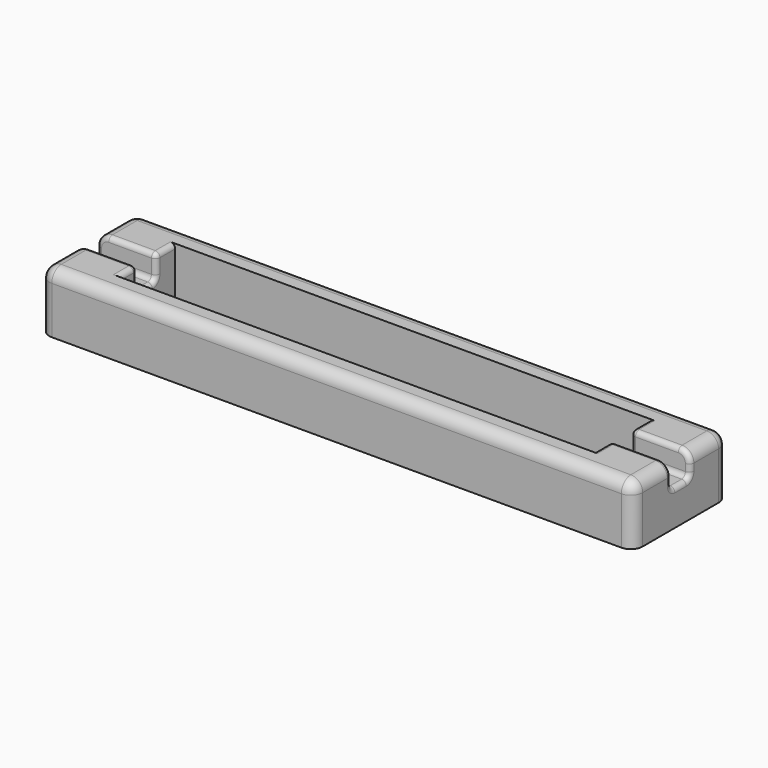
from build123d import *

# Parameters (mm, degrees)
F0_W         = 25
F0_H         = 5
F1_DEPTH     = 2.5
F2_W         = 20
F2_H         = 3
F3_DEPTH     = 2
F4_W         = 2.5
F4_H         = 1
F5_DEPTH     = 1
F6_F1_R      = 0.2
F6_F2_R      = 0.2
F7_T1_DEPTH  = 24
F7_T3_DEPTH  = 1.5
F7_T5_DEPTH  = 3.25
F7_T7_DEPTH  = 1.5
F7_T10_ANGLE = 90
F7_T12_ANGLE = 90
F7_T14_ANGLE = 90
F7_T16_ANGLE = 90
F7_S19_W     = 0.5
F7_S19_H     = 0.5
F7_T20_DEPTH = 0.5
F7_S25_W     = 0.5
F7_S25_H     = 0.5
F7_T26_DEPTH = 0.5
F7_S31_W     = 0.5
F7_S31_H     = 0.5
F7_T32_DEPTH = 0.5
F7_S37_W     = 0.5
F7_S37_H     = 0.5
F7_T38_DEPTH = 0.5


# Not quite as in the source:
# - a fillet or chamfer that OpenCascade refuses, or shapes differently, is made with other operations: its cross-section is extruded or revolved along the edge and cut away or added


with BuildPart() as f1:
    # F0 (on Top) → F1 (new body)
    with BuildSketch(Plane.XY):
        Rectangle(F0_W, F0_H)
    extrude(amount=F1_DEPTH)

    # F2 (on face) → F3 (cut)
    with BuildSketch(Plane.XY.offset(2.5)):
        Rectangle(F2_W, F2_H)
    extrude(amount=-F3_DEPTH, mode=Mode.SUBTRACT)

    # F4 (on face) → F5 (cut)
    with BuildSketch(Plane.XY.offset(2.5)):
        with Locations((-11.25, 0)):
            Rectangle(F4_W, F4_H)
        with Locations((11.25, 0)):
            Rectangle(F4_W, F4_H)
    extrude(amount=-F5_DEPTH, mode=Mode.SUBTRACT)

    # F6: fillet of radius 0.2 on 16 edges, made by hand

    # F6_f1
    f6_f1_edges = [f1.edges().sort_by_distance(p)[0] for p in [
        (-11.25, -0.5, 1.5),
        (-11.25, 0.5, 1.5),
        (11.25, -0.5, 1.5),
        (11.25, 0.5, 1.5),
    ]]
    fillet(f6_f1_edges, radius=F6_F1_R)

    # F6_f2
    f6_f2_edges = [f1.edges().sort_by_distance(p)[0] for p in [
        (-10, -0.5, 2.1),
        (10, 0, 1.5),
        (12.5, -0.5, 2.1),
        (-12.5, 0.5, 2.1),
        (-11.25, 0.5, 2.5),
        (-11.25, -0.5, 2.5),
        (11.25, 0.5, 2.5),
        (11.25, -0.5, 2.5),
        (-10, 1, 2.5),
        (10, 1, 2.5),
        (10, -1, 2.5),
        (-10, -1, 2.5),
        (-12.5, 0.4414213562, 1.5585786438),
        (12.5, -0.4414213562, 1.5585786438),
        (10, 0.4414213562, 1.5585786438),
        (10, -0.4414213562, 1.5585786438),
        (-10, -0.4414213562, 1.5585786438),
    ]]
    fillet(f6_f2_edges, radius=F6_F2_R)

    # F7: fillet of radius 0.5 on 10 edges, made by hand

    # F7_s2 → F7_t1 (cut)
    with BuildSketch(Plane.YZ.offset(-12)):
        with BuildLine():
            ThreePointArc((-2.5, 2), (-2.3535533906, 2.3535533906), (-2, 2.5))
            Line((-2, 2.5), (-2.5, 2.5))
            Line((-2.5, 2.5), (-2.5, 2))
        make_face()
        with BuildLine():
            ThreePointArc((2, 2.5), (2.3535533906, 2.3535533906), (2.5, 2))
            Line((2.5, 2), (2.5, 2.5))
            Line((2.5, 2.5), (2, 2.5))
        make_face()
    extrude(amount=F7_T1_DEPTH, mode=Mode.SUBTRACT)

    # F7_s4 → F7_t3 (cut)
    with BuildSketch(Plane.XZ.offset(0.5)):
        with BuildLine():
            ThreePointArc((-12, 2.5), (-12.3535533906, 2.3535533906), (-12.5, 2))
            Line((-12.5, 2), (-12.5, 2.5))
            Line((-12.5, 2.5), (-12, 2.5))
        make_face()
        with BuildLine():
            ThreePointArc((12.5, 2), (12.3535533906, 2.3535533906), (12, 2.5))
            Line((12, 2.5), (12.5, 2.5))
            Line((12.5, 2.5), (12.5, 2))
        make_face()
    extrude(amount=F7_T3_DEPTH, mode=Mode.SUBTRACT)

    # F7_s6 → F7_t5 (cut)
    with BuildSketch(Plane.XY.offset(-1.25)):
        with BuildLine():
            ThreePointArc((-12, -2.5), (-12.3535533906, -2.3535533906), (-12.5, -2))
            Line((-12.5, -2), (-12.5, -2.5))
            Line((-12.5, -2.5), (-12, -2.5))
        make_face()
        with BuildLine():
            ThreePointArc((12.5, -2), (12.3535533906, -2.3535533906), (12, -2.5))
            Line((12, -2.5), (12.5, -2.5))
            Line((12.5, -2.5), (12.5, -2))
        make_face()
        with BuildLine():
            ThreePointArc((-12, 2.5), (-12.3535533906, 2.3535533906), (-12.5, 2))
            Line((-12.5, 2), (-12.5, 2.5))
            Line((-12.5, 2.5), (-12, 2.5))
        make_face()
        with BuildLine():
            ThreePointArc((12.5, 2), (12.3535533906, 2.3535533906), (12, 2.5))
            Line((12, 2.5), (12.5, 2.5))
            Line((12.5, 2.5), (12.5, 2))
        make_face()
    extrude(amount=F7_T5_DEPTH, mode=Mode.SUBTRACT)

    # F7_s8 → F7_t7 (cut)
    with BuildSketch(Plane.XZ.offset(-2)):
        with BuildLine():
            ThreePointArc((-12, 2.5), (-12.3535533906, 2.3535533906), (-12.5, 2))
            Line((-12.5, 2), (-12.5, 2.5))
            Line((-12.5, 2.5), (-12, 2.5))
        make_face()
        with BuildLine():
            ThreePointArc((12.5, 2), (12.3535533906, 2.3535533906), (12, 2.5))
            Line((12, 2.5), (12.5, 2.5))
            Line((12.5, 2.5), (12.5, 2))
        make_face()
    extrude(amount=F7_T7_DEPTH, mode=Mode.SUBTRACT)

    # F7_s9 → F7_t10 (revolve, cut)
    with BuildSketch(Plane.XY.offset(2)):
        with BuildLine():
            ThreePointArc((12.3, 0.5), (12.4414213562, 0.5585786438), (12.5, 0.7))
            Line((12.5, 0.7), (12.5, 0.5))
            Line((12.5, 0.5), (12.3, 0.5))
        make_face()
    revolve(axis=Axis((12, 0.5, 2), (0, -1, 0)), revolution_arc=F7_T10_ANGLE, mode=Mode.SUBTRACT)

    # F7_s11 → F7_t12 (revolve, cut)
    with BuildSketch(Plane.YZ.offset(-12)):
        with BuildLine():
            ThreePointArc((0.5, 2.3), (0.5585786438, 2.4414213562), (0.7, 2.5))
            Line((0.7, 2.5), (0.5, 2.5))
            Line((0.5, 2.5), (0.5, 2.3))
        make_face()
    revolve(axis=Axis((-12, 0.5, 2), (0, -1, 0)), revolution_arc=F7_T12_ANGLE, mode=Mode.SUBTRACT)

    # F7_s13 → F7_t14 (revolve, cut)
    with BuildSketch(Plane.YZ.offset(12)):
        with BuildLine():
            ThreePointArc((-0.5, 2.3), (-0.5585786438, 2.4414213562), (-0.7, 2.5))
            Line((-0.7, 2.5), (-0.5, 2.5))
            Line((-0.5, 2.5), (-0.5, 2.3))
        make_face()
    revolve(axis=Axis((12, -0.5, 2), (0, 1, 0)), revolution_arc=F7_T14_ANGLE, mode=Mode.SUBTRACT)

    # F7_s15 → F7_t16 (revolve, cut)
    with BuildSketch(Plane.XY.offset(2)):
        with BuildLine():
            ThreePointArc((-12.3, -0.5), (-12.4414213562, -0.5585786438), (-12.5, -0.7))
            Line((-12.5, -0.7), (-12.5, -0.5))
            Line((-12.5, -0.5), (-12.3, -0.5))
        make_face()
    revolve(axis=Axis((-12, -0.5, 2), (0, 1, 0)), revolution_arc=F7_T16_ANGLE, mode=Mode.SUBTRACT)


with BuildPart() as f7_tool18:
    # F7_s19 → F7_t20 (new body)
    with BuildSketch(Plane.XY.offset(2)):
        with Locations((-12.25, -2.25)):
            Rectangle(F7_S19_W, F7_S19_H)
    extrude(amount=F7_T20_DEPTH)

    # F7_s21 → F7_t22 (revolve, cut)
    with BuildSketch(Plane(origin=(-12, -2, 2), x_dir=(0.7071067812, 0.7071067812, 0), z_dir=(0.7071067812, -0.7071067812, 0))):
        with BuildLine():
            ThreePointArc((0, -0.5), (0.5, 0), (0, 0.5))
            Line((0, 0.5), (0, -0.5))
        make_face()
    revolve(axis=Axis((-12, -2, 2), (0, 0, 1)), mode=Mode.SUBTRACT)


with BuildPart() as f1_1:
    add(f1.part)

    # F7_t17: cut F7_tool18
    add(f7_tool18.part, mode=Mode.SUBTRACT)


with BuildPart() as f7_tool24:
    # F7_s25 → F7_t26 (new body)
    with BuildSketch(Plane.YZ.offset(12)):
        with Locations((-2.25, 2.25)):
            Rectangle(F7_S25_W, F7_S25_H)
    extrude(amount=F7_T26_DEPTH)

    # F7_s27 → F7_t28 (revolve, cut)
    with BuildSketch(Plane(origin=(12, -2, 2), x_dir=(0, 0.7071067812, -0.7071067812), z_dir=(0, -0.7071067812, -0.7071067812))):
        with BuildLine():
            ThreePointArc((0, -0.5), (0.5, 0), (0, 0.5))
            Line((0, 0.5), (0, -0.5))
        make_face()
    revolve(axis=Axis((12, -2, 2), (1, 0, 0)), mode=Mode.SUBTRACT)


with BuildPart() as f1_2:
    add(f1_1.part)

    # F7_t23: cut F7_tool24
    add(f7_tool24.part, mode=Mode.SUBTRACT)


with BuildPart() as f7_tool30:
    # F7_s31 → F7_t32 (new body)
    with BuildSketch(Plane.YZ.offset(12)):
        with Locations((2.25, 2.25)):
            Rectangle(F7_S31_W, F7_S31_H)
    extrude(amount=F7_T32_DEPTH)

    # F7_s33 → F7_t34 (revolve, cut)
    with BuildSketch(Plane(origin=(12, 2, 2), x_dir=(0, -0.7071067812, -0.7071067812), z_dir=(0, -0.7071067812, 0.7071067812))):
        with BuildLine():
            ThreePointArc((0, -0.5), (0.5, 0), (0, 0.5))
            Line((0, 0.5), (0, -0.5))
        make_face()
    revolve(axis=Axis((12, 2, 2), (1, 0, 0)), mode=Mode.SUBTRACT)


with BuildPart() as f1_3:
    add(f1_2.part)

    # F7_t29: cut F7_tool30
    add(f7_tool30.part, mode=Mode.SUBTRACT)


with BuildPart() as f7_tool36:
    # F7_s37 → F7_t38 (new body)
    with BuildSketch(Plane.YZ.offset(-12)):
        with Locations((2.25, 2.25)):
            Rectangle(F7_S37_W, F7_S37_H)
    extrude(amount=-F7_T38_DEPTH)

    # F7_s39 → F7_t40 (revolve, cut)
    with BuildSketch(Plane(origin=(-12, 2, 2), x_dir=(0, -0.7071067812, -0.7071067812), z_dir=(0, 0.7071067812, -0.7071067812))):
        with BuildLine():
            ThreePointArc((0, -0.5), (0.5, 0), (0, 0.5))
            Line((0, 0.5), (0, -0.5))
        make_face()
    revolve(axis=Axis((-12, 2, 2), (-1, 0, 0)), mode=Mode.SUBTRACT)


with BuildPart() as f1_4:
    add(f1_3.part)

    # F7_t35: cut F7_tool36
    add(f7_tool36.part, mode=Mode.SUBTRACT)


solid = f1_4.part
